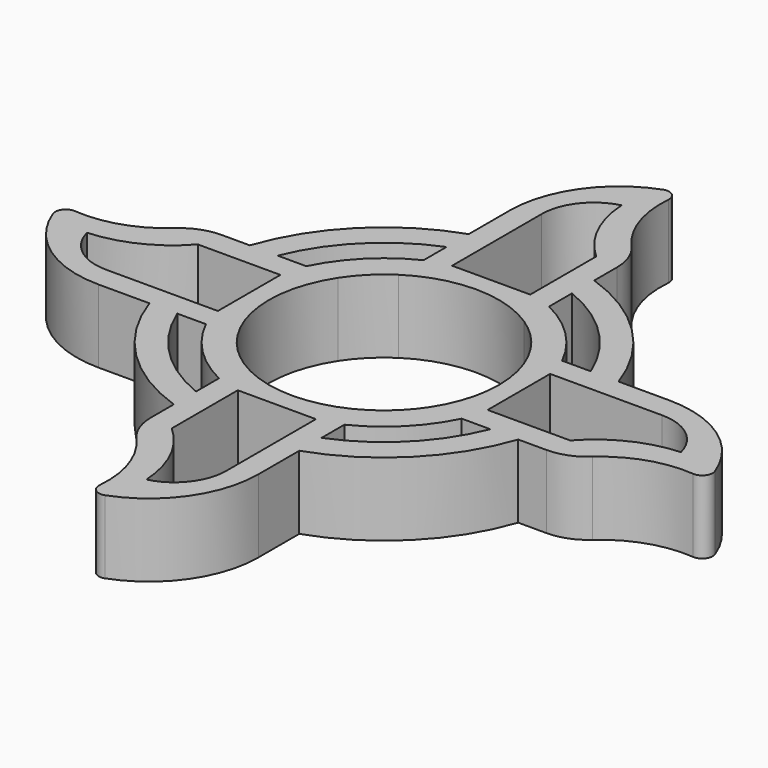
from build123d import *

# Parameters (mm, degrees)
F1_DEPTH = 7
F2_R     = 1
F3_R     = 5
F5_DEPTH = 25


# Not quite as in the source:
# - a feature names something its author has since deleted; it is built from what else it names


with BuildPart() as f1:
    # F0 (on Top) → F1 (new body)
    with BuildSketch(Plane.XY):
        with BuildLine():
            ThreePointArc((6, 14.9671515326), (11.4020968466, 11.4020968466), (14.9671515326, 6))
            Line((14.9671515326, 6), (17.6320907722, 6))
            ThreePointArc((17.6320907722, 6), (13.1698637996, 13.1698637996), (6, 17.6320907722))
            Line((6, 17.6320907722), (6, 14.9671515326))
        make_face()
        with BuildLine():
            Line((17.6320907722, 6), (14.9671515326, 6))
            ThreePointArc((14.9671515326, 6), (15.8328920836, 3.0553483056), (16.125, 0))
            ThreePointArc((16.125, 0), (15.8328920836, -3.0553483056), (14.9671515326, -6))
            Line((14.9671515326, -6), (17.6320907722, -6))
            ThreePointArc((17.6320907722, -6), (18.3750961308, -3.0408004183), (18.625, 0))
            ThreePointArc((18.625, 0), (18.3750961308, 3.0408004183), (17.6320907722, 6))
        make_face()
        with BuildLine():
            Line((17.6320907722, -6), (14.9671515326, -6))
            ThreePointArc((14.9671515326, -6), (11.4020968466, -11.4020968466), (6, -14.9671515326))
            Line((6, -14.9671515326), (6, -17.6320907722))
            ThreePointArc((6, -17.6320907722), (13.1698637996, -13.1698637996), (17.6320907722, -6))
        make_face()
        with BuildLine():
            ThreePointArc((-6, 14.9671515326), (0, 16.125), (6, 14.9671515326))
            Line((6, 14.9671515326), (6, 17.6320907722))
            ThreePointArc((6, 17.6320907722), (0, 18.625), (-6, 17.6320907722))
            Line((-6, 17.6320907722), (-6, 14.9671515326))
        make_face()
        with BuildLine():
            Line((22.5, 6), (17.6320907722, 6))
            ThreePointArc((17.6320907722, 6), (18.3750961308, 3.0408004183), (18.625, 0))
            ThreePointArc((18.625, 0), (18.3750961308, -3.0408004183), (17.6320907722, -6))
            Line((17.6320907722, -6), (22.5, -6))
            Line((22.5, -6), (22.5, 6))
        make_face()
        with BuildLine():
            Line((6, -17.6320907722), (6, -14.9671515326))
            ThreePointArc((6, -14.9671515326), (0, -16.125), (-6, -14.9671515326))
            Line((-6, -14.9671515326), (-6, -17.6320907722))
            ThreePointArc((-6, -17.6320907722), (0, -18.625), (6, -17.6320907722))
        make_face()
        with BuildLine():
            ThreePointArc((-14.9671515326, 6), (-11.4020968466, 11.4020968466), (-6, 14.9671515326))
            Line((-6, 14.9671515326), (-6, 17.6320907722))
            ThreePointArc((-6, 17.6320907722), (-13.1698637996, 13.1698637996), (-17.6320907722, 6))
            Line((-17.6320907722, 6), (-14.9671515326, 6))
        make_face()
        with BuildLine():
            ThreePointArc((-6, 17.6320907722), (0, 18.625), (6, 17.6320907722))
            Line((6, 17.6320907722), (6, 22.5))
            Line((6, 22.5), (-6, 22.5))
            Line((-6, 22.5), (-6, 17.6320907722))
        make_face()
        with BuildLine():
            ThreePointArc((32.757434994, -2.4008296896), (29.1292705505, 3.631764353), (22.5, 6))
            Line((22.5, 6), (22.5, -6))
            ThreePointArc((22.5, -6), (27.1011186164, -2.6967874102), (32.757434994, -2.4008296896))
        make_face()
        with BuildLine():
            Line((-6, -17.6320907722), (-6, -14.9671515326))
            ThreePointArc((-6, -14.9671515326), (-11.4020968466, -11.4020968466), (-14.9671515326, -6))
            Line((-14.9671515326, -6), (-17.6320907722, -6))
            ThreePointArc((-17.6320907722, -6), (-13.1698637996, -13.1698637996), (-6, -17.6320907722))
        make_face()
        with BuildLine():
            Line((6, -22.5), (6, -17.6320907722))
            ThreePointArc((6, -17.6320907722), (0, -18.625), (-6, -17.6320907722))
            Line((-6, -17.6320907722), (-6, -22.5))
            Line((-6, -22.5), (6, -22.5))
        make_face()
        with BuildLine():
            ThreePointArc((-14.9671515326, -6), (-16.125, 0), (-14.9671515326, 6))
            Line((-14.9671515326, 6), (-17.6320907722, 6))
            ThreePointArc((-17.6320907722, 6), (-18.625, 0), (-17.6320907722, -6))
            Line((-17.6320907722, -6), (-14.9671515326, -6))
        make_face()
        with BuildLine():
            Line((-6, 22.5), (6, 22.5))
            ThreePointArc((6, 22.5), (2.6967874102, 27.1011186164), (2.4008296896, 32.757434994))
            ThreePointArc((2.4008296896, 32.757434994), (-3.631764353, 29.1292705505), (-6, 22.5))
        make_face()
        with BuildLine():
            ThreePointArc((-2.4008296896, -32.757434994), (3.631764353, -29.1292705505), (6, -22.5))
            Line((6, -22.5), (-6, -22.5))
            ThreePointArc((-6, -22.5), (-2.6967874102, -27.1011186164), (-2.4008296896, -32.757434994))
        make_face()
        with BuildLine():
            ThreePointArc((-17.6320907722, -6), (-18.625, 0), (-17.6320907722, 6))
            Line((-17.6320907722, 6), (-22.5, 6))
            Line((-22.5, 6), (-22.5, -6))
            Line((-22.5, -6), (-17.6320907722, -6))
        make_face()
        with BuildLine():
            Line((-22.5, -6), (-22.5, 6))
            ThreePointArc((-22.5, 6), (-27.1011186164, 2.6967874102), (-32.757434994, 2.4008296896))
            ThreePointArc((-32.757434994, 2.4008296896), (-29.1292705505, -3.631764353), (-22.5, -6))
        make_face()
        with BuildLine():
            ThreePointArc((-6, 12.2327684929), (0, 13.625), (6, 12.2327684929))
            Line((6, 12.2327684929), (6, 14.9671515326))
            ThreePointArc((6, 14.9671515326), (0, 16.125), (-6, 14.9671515326))
            Line((-6, 14.9671515326), (-6, 12.2327684929))
        make_face()
        with BuildLine():
            ThreePointArc((-6, 9.2195444573), (0, 11), (6, 9.2195444573))
            Line((6, 9.2195444573), (6, 12.2327684929))
            ThreePointArc((6, 12.2327684929), (0, 13.625), (-6, 12.2327684929))
            Line((-6, 12.2327684929), (-6, 9.2195444573))
        make_face()
        with BuildLine():
            ThreePointArc((-12.2327684929, -6), (-13.625, 0), (-12.2327684929, 6))
            Line((-12.2327684929, 6), (-14.9671515326, 6))
            ThreePointArc((-14.9671515326, 6), (-16.125, 0), (-14.9671515326, -6))
            Line((-14.9671515326, -6), (-12.2327684929, -6))
        make_face()
        with BuildLine():
            ThreePointArc((-9.2195444573, -6), (-11, 0), (-9.2195444573, 6))
            Line((-9.2195444573, 6), (-12.2327684929, 6))
            ThreePointArc((-12.2327684929, 6), (-13.625, 0), (-12.2327684929, -6))
            Line((-12.2327684929, -6), (-9.2195444573, -6))
        make_face()
        with BuildLine():
            Line((14.9671515326, 6), (12.2327684929, 6))
            ThreePointArc((12.2327684929, 6), (13.2723791333, 3.0797040673), (13.625, 0))
            ThreePointArc((13.625, 0), (13.2723791333, -3.0797040673), (12.2327684929, -6))
            Line((12.2327684929, -6), (14.9671515326, -6))
            ThreePointArc((14.9671515326, -6), (15.8328920836, -3.0553483056), (16.125, 0))
            ThreePointArc((16.125, 0), (15.8328920836, 3.0553483056), (14.9671515326, 6))
        make_face()
        with BuildLine():
            ThreePointArc((9.2195444573, 6), (10.5454964091, 3.129297922), (11, 0))
            ThreePointArc((11, 0), (10.5454964091, -3.129297922), (9.2195444573, -6))
            Line((9.2195444573, -6), (12.2327684929, -6))
            ThreePointArc((12.2327684929, -6), (13.2723791333, -3.0797040673), (13.625, 0))
            ThreePointArc((13.625, 0), (13.2723791333, 3.0797040673), (12.2327684929, 6))
            Line((12.2327684929, 6), (9.2195444573, 6))
        make_face()
        with BuildLine():
            Line((6, -14.9671515326), (6, -12.2327684929))
            ThreePointArc((6, -12.2327684929), (0, -13.625), (-6, -12.2327684929))
            Line((-6, -12.2327684929), (-6, -14.9671515326))
            ThreePointArc((-6, -14.9671515326), (0, -16.125), (6, -14.9671515326))
        make_face()
        with BuildLine():
            Line((6, -12.2327684929), (6, -9.2195444573))
            ThreePointArc((6, -9.2195444573), (0, -11), (-6, -9.2195444573))
            Line((-6, -9.2195444573), (-6, -12.2327684929))
            ThreePointArc((-6, -12.2327684929), (0, -13.625), (6, -12.2327684929))
        make_face()
        with BuildLine():
            ThreePointArc((-9.2195444573, 6), (-7.7781745931, 7.7781745931), (-6, 9.2195444573))
            Line((-6, 9.2195444573), (-6, 12.2327684929))
            ThreePointArc((-6, 12.2327684929), (-9.6343298937, 9.6343298937), (-12.2327684929, 6))
            Line((-12.2327684929, 6), (-9.2195444573, 6))
        make_face()
        with BuildLine():
            ThreePointArc((6, 9.2195444573), (7.7781745931, 7.7781745931), (9.2195444573, 6))
            Line((9.2195444573, 6), (12.2327684929, 6))
            ThreePointArc((12.2327684929, 6), (9.6343298937, 9.6343298937), (6, 12.2327684929))
            Line((6, 12.2327684929), (6, 9.2195444573))
        make_face()
        with BuildLine():
            Line((12.2327684929, -6), (9.2195444573, -6))
            ThreePointArc((9.2195444573, -6), (7.7781745931, -7.7781745931), (6, -9.2195444573))
            Line((6, -9.2195444573), (6, -12.2327684929))
            ThreePointArc((6, -12.2327684929), (9.6343298937, -9.6343298937), (12.2327684929, -6))
        make_face()
        with BuildLine():
            Line((-6, -12.2327684929), (-6, -9.2195444573))
            ThreePointArc((-6, -9.2195444573), (-7.7781745931, -7.7781745931), (-9.2195444573, -6))
            Line((-9.2195444573, -6), (-12.2327684929, -6))
            ThreePointArc((-12.2327684929, -6), (-9.6343298937, -9.6343298937), (-6, -12.2327684929))
        make_face()
    extrude(amount=F1_DEPTH)

    # F2
    f2_edges = [f1.edges().sort_by_distance(p)[0] for p in [
        (-2.40083, -32.757435, 3.5),
        (-32.757435, 2.40083, 3.5),
        (32.757435, -2.40083, 3.5),
        (2.40083, 32.757435, 3.5),
    ]]
    fillet(f2_edges, radius=F2_R)

    # F3
    f3_edges = [f1.edges().sort_by_distance(p)[0] for p in [
        (-22.5, 6, 3.5),
        (6, 22.5, 3.5),
        (22.5, -6, 3.5),
        (-6, -22.5, 3.5),
    ]]
    fillet(f3_edges, radius=F3_R)

    # F4 (on face) → F5 (cut)
    with BuildSketch(Plane.XY.offset(7)):
        with BuildLine():
            ThreePointArc((0, 28.4005012363), (-2.7218256359, 26.630820183), (-3.7782429717, 23.5609523952))
            Line((-3.7782429717, 23.5609523952), (-3.7782429717, 12.8630073741))
            Line((-3.7782429717, 12.8630073741), (3.6933382507, 12.8630073741))
            Line((3.6933382507, 12.8630073741), (3.6933382507, 20.7591112703))
            ThreePointArc((3.6933382507, 20.7591112703), (1.0835977394, 24.21098844), (0, 28.4005012363))
        make_face()
        with BuildLine():
            ThreePointArc((-20.7591112703, 3.6933382507), (-24.21098844, 1.0835977394), (-28.4005012363, 0))
            ThreePointArc((-28.4005012363, 0), (-26.630820183, -2.7218256359), (-23.5609523952, -3.7782429717))
            Line((-23.5609523952, -3.7782429717), (-12.8630073741, -3.7782429717))
            Line((-12.8630073741, -3.7782429717), (-12.8630073741, 3.6933382507))
            Line((-12.8630073741, 3.6933382507), (-20.7591112703, 3.6933382507))
        make_face()
        with BuildLine():
            ThreePointArc((-3.6933382507, -20.7591112703), (-1.0835977394, -24.21098844), (0, -28.4005012363))
            ThreePointArc((0, -28.4005012363), (2.7218256359, -26.630820183), (3.7782429717, -23.5609523952))
            Line((3.7782429717, -23.5609523952), (3.7782429717, -12.8630073741))
            Line((3.7782429717, -12.8630073741), (-3.6933382507, -12.8630073741))
            Line((-3.6933382507, -12.8630073741), (-3.6933382507, -20.7591112703))
        make_face()
        with BuildLine():
            ThreePointArc((20.7591112703, -3.6933382507), (24.21098844, -1.0835977394), (28.4005012363, 0))
            ThreePointArc((28.4005012363, 0), (26.630820183, 2.7218256359), (23.5609523952, 3.7782429717))
            Line((23.5609523952, 3.7782429717), (12.8630073741, 3.7782429717))
            Line((12.8630073741, 3.7782429717), (12.8630073741, -3.6933382507))
            Line((12.8630073741, -3.6933382507), (20.7591112703, -3.6933382507))
        make_face()
    extrude(amount=-F5_DEPTH, mode=Mode.SUBTRACT)


solid = f1.part
